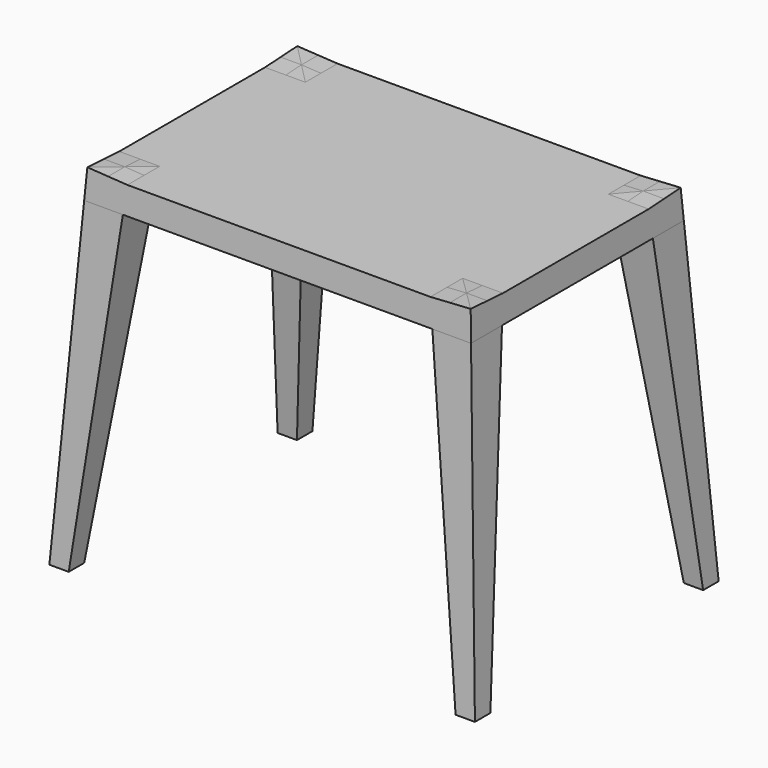
from build123d import *

# Parameters (mm, degrees)
F1_DEPTH = 558.8
F2_DEPTH = 558.8
F4_DEPTH = 400.051
F5_DEPTH = 400.051


with BuildPart() as f1:
    # F0 (on Right) → F1 (new body)
    with BuildSketch(Plane.YZ):
        Polygon((-50.6140871806, 419.1), (-25.4, 419.1), (-27.7090909091, 457.2), (-55.0315530236, 455.5440932052), align=None)
        Polygon((-76.2, 419.1), (-50.6140871806, 419.1), (-55.0315530236, 455.5440932052), (-80.4308776001, 454.0047402005), align=None)
        Polygon((-323.85, 419.1), (-76.2, 419.1), (-80.4308776001, 454.0047402005), (-319.6191223999, 454.0047402005), align=None)
        Polygon((-349.4359128194, 419.1), (-323.85, 419.1), (-319.6191223999, 454.0047402005), (-345.0184469764, 455.5440932052), align=None)
        Polygon((-374.65, 419.1), (-349.4359128194, 419.1), (-345.0184469764, 455.5440932052), (-372.3409090909, 457.2), align=None)
    extrude(amount=F1_DEPTH)


with BuildPart() as f2:
    # F0 (on Right) → F2 (new body, through all)
    with BuildSketch(Plane.YZ):
        Polygon((-25.4, 0), (0, 0), (-25.4, 419.1), (-50.6140871806, 419.1), (-76.2, 419.1), align=None)
        Polygon((-76.2, 419.1), (-50.6140871806, 419.1), (-55.0315530236, 455.5440932052), (-80.4308776001, 454.0047402005), align=None)
    extrude(amount=F2_DEPTH)


with BuildPart() as f2b:
    # F0 (on Right) → F2, piece 2 (new body, through all)
    with BuildSketch(Plane.YZ):
        Polygon((-374.65, 0), (-323.85, 419.1), (-349.4359128194, 419.1), (-374.65, 419.1), (-400.05, 0), align=None)
        Polygon((-349.4359128194, 419.1), (-323.85, 419.1), (-319.6191223999, 454.0047402005), (-345.0184469764, 455.5440932052), align=None)
    extrude(amount=F2_DEPTH)


with BuildPart() as f4_tool:
    # F3 (on Front) → F4 (new body, through all)
    with BuildSketch(Plane.XZ):
        Polygon((25.4, 0), (533.4, 0), (482.6, 419.1), (76.2, 419.1), align=None)
        Polygon((503.7684469764, 455.5440932052), (531.0909090909, 457.2), (27.7090909091, 457.2), (55.0315530236, 455.5440932052), (80.4308776001, 454.0047402005), (478.3691223999, 454.0047402005), align=None)
        Polygon((533.4, 419.1), (558.8, 0), (558.8, 457.2), (531.0909090909, 457.2), align=None)
        Polygon((25.4, 419.1), (27.7090909091, 457.2), (0, 457.2), (0, 0), align=None)
    extrude(amount=F4_DEPTH)


with BuildPart() as f1_1:
    add(f1.part)

    # F4: cut by f4_tool
    add(f4_tool.part, mode=Mode.SUBTRACT)


with BuildPart() as f2_1:
    add(f2.part)

    # F4: cut by f4_tool
    add(f4_tool.part, mode=Mode.SUBTRACT)


with BuildPart() as f2b_1:
    add(f2b.part)

    # F4: cut by f4_tool
    add(f4_tool.part, mode=Mode.SUBTRACT)


with BuildPart() as f5_tool:
    # F3 (on Front) → F5 (new body, through all)
    with BuildSketch(Plane.XZ):
        Polygon((508.1859128194, 419.1), (533.4, 419.1), (531.0909090909, 457.2), (503.7684469764, 455.5440932052), align=None)
        Polygon((55.0315530236, 455.5440932052), (27.7090909091, 457.2), (25.4, 419.1), (50.6140871806, 419.1), align=None)
        Polygon((76.2, 419.1), (482.6, 419.1), (478.3691223999, 454.0047402005), (80.4308776001, 454.0047402005), align=None)
    extrude(amount=F5_DEPTH)


with BuildPart() as f2_2:
    add(f2_1.part)

    # F5: cut by f5_tool
    add(f5_tool.part, mode=Mode.SUBTRACT)


with BuildPart() as f2b_2:
    add(f2b_1.part)

    # F5: cut by f5_tool
    add(f5_tool.part, mode=Mode.SUBTRACT)


with BuildPart() as f1_2:
    add(f1_1.part)

    # F6: cut F2b, F2
    add(f2b_2.part, mode=Mode.SUBTRACT)
    add(f2_2.part, mode=Mode.SUBTRACT)


solid = Compound([f2_2.part, f2b_2.part, f1_2.part])
